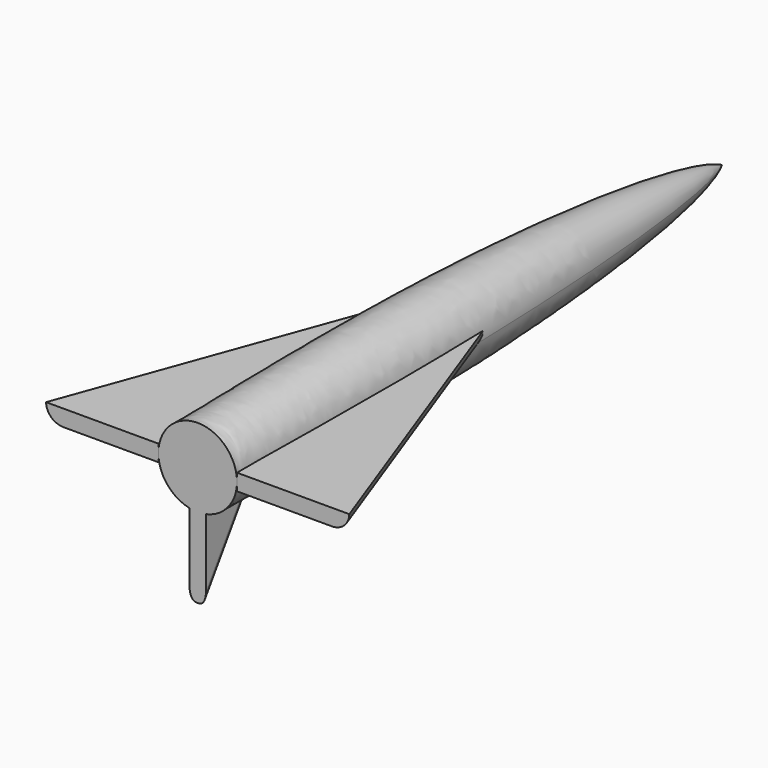
from build123d import *

# Parameters (mm, degrees)
F2_DEPTH = 2.5
F3_R     = 4.99999
F6_DEPTH = 2.5
F7_R     = 2
F8_R     = 2


# Not quite as in the source:
# - a fillet or chamfer is up to 0.001 mm smaller than in the source, because OpenCascade refuses the exact size


with BuildPart() as f1:
    # F0 (on Top) → F1 (revolve)
    with BuildSketch(Plane.XY):
        with BuildLine():
            Line((0, 200), (0, 0))
            Line((0, 0), (12, 0))
            add(Edge.make_bspline(
                [(12, 0), (11.666193583, 5.5268802411), (13.2381964863, 49.5672633882), (12, 93.9436979115)],
                knots=[0, 0, 0, 0, 0.484051037, 0.484051037, 0.484051037, 0.484051037], degree=3))
            add(Edge.make_bspline(
                [(12, 93.9436979115), (10.6802090187, 141.2444443711), (6.1676430445, 188.9269916502), (0, 200)],
                knots=[0.484051037, 0.484051037, 0.484051037, 0.484051037, 1, 1, 1, 1], degree=3))
        make_face()
    revolve(axis=Axis((0, 100, 0), (0, 1, 0)))

    # F0 (on Top) → F2 (join, symmetric)
    with BuildSketch(Plane.XY):
        with BuildLine():
            add(Edge.make_bspline(
                [(12, 0), (11.666193583, 5.5268802411), (13.2381964863, 49.5672633882), (12, 93.9436979115)],
                knots=[0, 0, 0, 0, 0.484051037, 0.484051037, 0.484051037, 0.484051037], degree=3))
            Line((12, 0), (46.2721697986, 0))
            Line((46.2721697986, 0), (12, 93.9436979115))
        make_face()
    extrude(amount=F2_DEPTH, both=True)

    # F3 (radius 5 in the source; OpenCascade refuses exactly that, so slightly less here)
    f3_edges = [f1.edges().sort_by_distance(p)[0] for p in [
        (29.136085, 46.971849, -2.5),
    ]]
    fillet(f3_edges, radius=F3_R)

    # F4: F1 across plane


with BuildPart() as f1_1:
    add(f1.part)
    add(f1.part.mirror(Plane.YZ))

    # F5 (on Right) → F6 (join, symmetric)
    with BuildSketch(Plane.YZ):
        Polygon((20, -6.398999393), (0, -6.398999393), (0, -36.398999393), align=None)
    extrude(amount=F6_DEPTH, both=True)

    # F7
    f7_edges = [f1_1.edges().sort_by_distance(p)[0] for p in [
        (2.5, 8.180642, -24.128037),
    ]]
    fillet(f7_edges, radius=F7_R)

    # F8
    f8_edges = [f1_1.edges().sort_by_distance(p)[0] for p in [
        (-2.5, 8.180642, -24.128037),
    ]]
    fillet(f8_edges, radius=F8_R)


solid = f1_1.part
